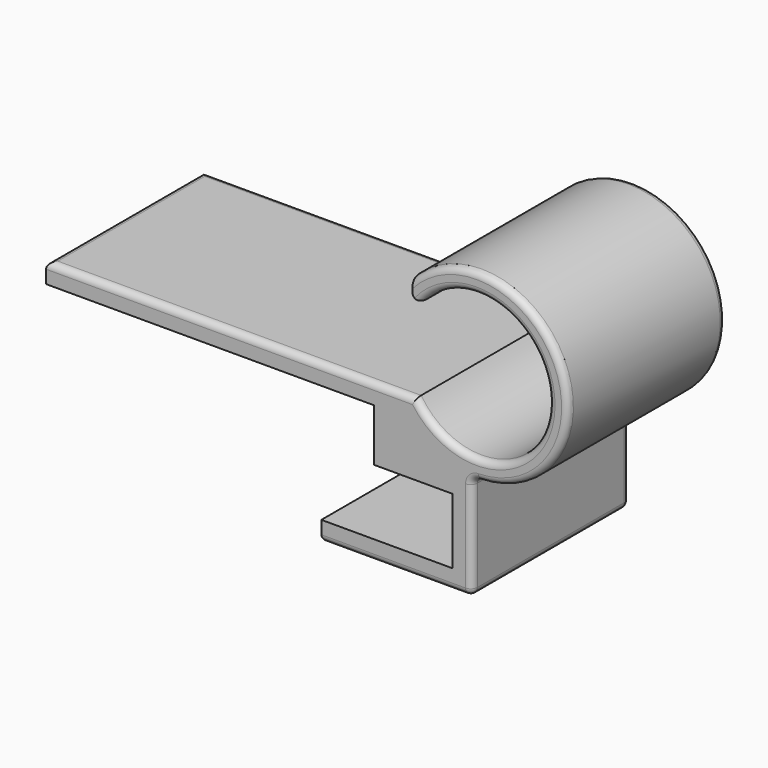
from build123d import *

# Parameters (mm, degrees)
F0_W          = 50
F0_H          = 3
F0_W_2        = 3
F0_W_3        = 9
F0_H_2        = 10
F1_DEPTH      = 15
F1_DEPTH_BACK = 15
F2_R          = 1


with BuildPart() as f1:
    # F0 (on Front) → F1 (new body, two sides)
    with BuildSketch(Plane.XZ) as f1_sk:
        with Locations((25, 1.5)):
            Rectangle(F0_W, F0_H)
        Polygon((50, 3), (50, 0), (50, -5), (53, -5), (53, 3), align=None)
        with Locations((51.5, -6.5)):
            Rectangle(F0_W_2, F0_H)
        with BuildLine():
            ThreePointArc((65, -5), (57.8905996075, -2.6641005887), (53, 3))
            Line((53, 3), (53, -5))
            Line((53, -5), (62, -5))
            Line((62, -5), (65, -5))
        make_face()
        with BuildLine():
            Line((55.8741820756, 3), (53, 3))
            ThreePointArc((53, 3), (57.8905996075, -2.6641005887), (65, -5))
            ThreePointArc((65, -5), (78.7423188539, 13.9604240048), (55.8741820756, 19))
            Line((55.8741820756, 19), (55.8741820756, 14.0153257874))
            ThreePointArc((55.8741820756, 14.0153257874), (76.6425830118, 9.5358154417), (56.4268562898, 3))
            Line((56.4268562898, 3), (55.8741820756, 3))
        make_face()
        with Locations((57.5, -6.5)):
            Rectangle(F0_W_3, F0_H)
        with Locations((63.5, -6.5)):
            Rectangle(F0_W_2, F0_H)
        with Locations((63.5, -13)):
            Rectangle(F0_W_2, F0_H_2)
        Polygon((65, -21), (65, -18), (62, -18), (42, -18), (42, -21), align=None)
    extrude(amount=F1_DEPTH)
    extrude(f1_sk.sketch, amount=-F1_DEPTH_BACK)

    # F2
    f2_edges = [f1.edges().sort_by_distance(p)[0] for p in [
        (55.874182, 0, 14.015326),
        (65, 0, -21),
        (0, 0, 3),
        (78.742319, -15, 13.960424),
        (55.874182, 0, 19),
        (78.742319, 15, 13.960424),
        (65, 0, -5),
        (28.213428, 15, 3),
        (28.213428, -15, 3),
        (76.642583, -15, 9.535815),
        (76.642583, 15, 9.535815),
        (53.5, -15, -21),
        (53.5, 15, -21),
        (42, 0, -21),
        (65, 15, -13),
        (65, -15, -13),
    ]]
    fillet(f2_edges, radius=F2_R)


solid = f1.part
